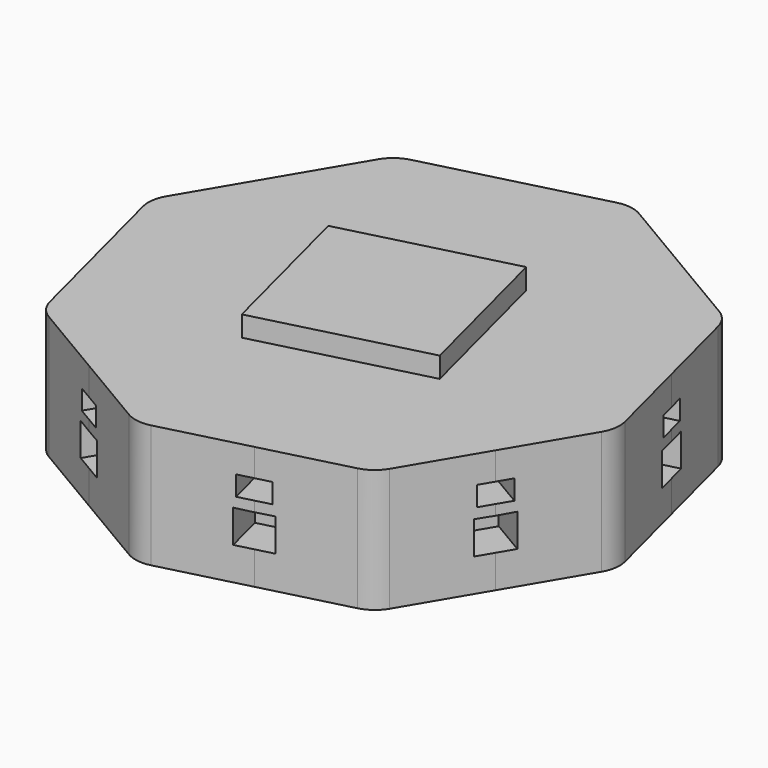
from build123d import *

# Parameters (mm, degrees)
F1_DEPTH  = 9.525
F3_DEPTH  = 6.35
F5_DEPTH  = 6.35
F7_DEPTH  = 6.35
F9_DEPTH  = 6.35
F11_DEPTH = 6.35
F13_DEPTH = 6.35
F15_DEPTH = 6.35
F17_DEPTH = 6.35
F19_DEPTH = 3.175
F20_R     = 5.08


# Not quite as in the source:
# - a feature names something its author has since deleted; it is built from what else it names


with BuildPart() as f1:
    # F0 (on Top) → F1 (new body, symmetric)
    with BuildSketch(Plane.XY):
        Polygon((-32.7905689314, 19.40073682), (-40.8266172422, 5.8184384507), (-36.9048262157, -9.4680410849), (0, 0), align=None)
        Polygon((-24.7545206205, 32.9830351893), (-32.7905689314, 19.40073682), (0, 0), (-9.4680410849, 36.9048262157), align=None)
        Polygon((-9.4680410849, 36.9048262157), (0, 0), (19.40073682, 32.7905689314), (5.8184384507, 40.8266172422), align=None)
        Polygon((19.40073682, 32.7905689314), (0, 0), (36.9048262157, 9.4680410849), (32.9830351893, 24.7545206205), align=None)
        Polygon((36.9048262157, 9.4680410849), (0, 0), (32.7905689314, -19.40073682), (40.8266172422, -5.8184384507), align=None)
        Polygon((32.7905689314, -19.40073682), (0, 0), (9.4680410849, -36.9048262157), (24.7545206205, -32.9830351893), align=None)
        Polygon((9.4680410849, -36.9048262157), (0, 0), (-19.40073682, -32.7905689314), (-5.8184384507, -40.8266172422), align=None)
        Polygon((0, 0), (-36.9048262157, -9.4680410849), (-32.9830351893, -24.7545206205), (-19.40073682, -32.7905689314), align=None)
    extrude(amount=F1_DEPTH, both=True)

    # F2 (on face) → F3 (cut)
    with BuildSketch(Plane(origin=(-36.9048262157, -9.4680410849, 0), x_dir=(0.2485050154, -0.9686306093, 0), z_dir=(-0.9686306093, -0.2485050154, 0))):
        Polygon((-2.794, 0), (-2.794, -2.521839), (-2.794, -5.043678), (2.794, -5.043678), (2.794, -2.521839), (2.794, 0), align=None)
        Polygon((-2.413, 1.556766), (0, 1.556766), (2.413, 1.556766), (2.413, 4.604766), (-2.413, 4.604766), align=None)
    extrude(amount=-F3_DEPTH, mode=Mode.SUBTRACT)

    # F4 (on face) → F5 (cut)
    with BuildSketch(Plane(origin=(-9.4680410849, 36.9048262157, 0), x_dir=(-0.9686306093, -0.2485050154, 0), z_dir=(-0.2485050154, 0.9686306093, 0))):
        Polygon((-2.794, -5.043678), (0, -5.043678), (2.794, -5.043678), (2.794, 0.036322), (0, 0), (-2.794, 0.036322), align=None)
        Polygon((-2.413, 1.593088), (0, 1.593088), (2.413, 1.593088), (2.413, 4.641088), (0, 4.641088), (-2.413, 4.641088), align=None)
    extrude(amount=-F5_DEPTH, mode=Mode.SUBTRACT)

    # F6 (on face) → F7 (cut)
    with BuildSketch(Plane(origin=(-32.7905689314, 19.40073682, 0), x_dir=(-0.5092056908, -0.8606448538, 0), z_dir=(-0.8606448538, 0.5092056908, 0))):
        Polygon((-2.413, 1.593088), (0, 1.593088), (2.413, 1.593088), (2.413, 4.641088), (0, 4.641088), (-2.413, 4.641088), align=None)
        Polygon((-2.794, -5.043678), (0, -5.043678), (2.794, -5.043678), (2.793763897, 0), (-2.793763897, 0), align=None)
    extrude(amount=-F7_DEPTH, mode=Mode.SUBTRACT)

    # F8 (on face) → F9 (cut)
    with BuildSketch(Plane(origin=(19.40073682, 32.7905689314, 0), x_dir=(-0.8606448538, 0.5092056908, 0), z_dir=(0.5092056908, 0.8606448538, 0))):
        Polygon((-2.413, 1.62941), (0, 1.62941), (2.413, 1.62941), (2.413, 4.67741), (-2.413, 4.67741), align=None)
        Polygon((-2.794, -5.043678), (0, -5.043678), (2.794, -5.043678), (2.794, 0.036322), (-2.794, 0.036322), align=None)
    extrude(amount=-F9_DEPTH, mode=Mode.SUBTRACT)

    # F10 (on face) → F11 (cut)
    with BuildSketch(Plane(origin=(36.9048262157, 9.4680410849, 0), x_dir=(-0.2485050154, 0.9686306093, 0), z_dir=(0.9686306093, 0.2485050154, 0))):
        Polygon((-2.794, -4.6912106667), (0, -4.6912106667), (2.794, -4.6912106667), (2.794, 0.3887893333), (-2.794, 0.3887893333), align=None)
        Polygon((-2.413, 1.9818773333), (0, 1.9818773333), (2.413, 1.9818773333), (2.413, 5.0298773333), (-2.413, 5.0298773333), align=None)
    extrude(amount=-F11_DEPTH, mode=Mode.SUBTRACT)

    # F12 (on face) → F13 (cut)
    with BuildSketch(Plane(origin=(32.7905689314, -19.40073682, 0), x_dir=(0.5092056908, 0.8606448538, 0), z_dir=(0.8606448538, -0.5092056908, 0))):
        Polygon((-2.7940002649, -4.4215812), (-2.649e-07, -4.4215812), (2.7939997351, -4.4215812), (2.7939997351, 0.6584188), (-2.649e-07, 0.6220968), (-2.7940002649, 0.6584188), align=None)
        Polygon((-2.4130002649, 2.2151848), (-2.649e-07, 2.2151848), (2.4129997351, 2.2151848), (2.4129997351, 5.2631848), (-2.649e-07, 5.2631848), (-2.4130002649, 5.2631848), align=None)
    extrude(amount=-F13_DEPTH, mode=Mode.SUBTRACT)

    # F14 (on face) → F15 (cut)
    with BuildSketch(Plane(origin=(9.4680410849, -36.9048262157, 0), x_dir=(0.9686306093, 0.2485050154, 0), z_dir=(0.2485050154, -0.9686306093, 0))):
        Polygon((-2.7940002649, -4.4215812), (-2.649e-07, -4.4215812), (2.7939997351, -4.4215812), (2.7939997351, 0.6584188), (-2.649e-07, 0.6220968), (-2.7940002649, 0.6584188), align=None)
        Polygon((-2.4130002649, 2.2151848), (-2.649e-07, 2.2151848), (2.4129997351, 2.2151848), (2.4129997351, 5.2631848), (-2.649e-07, 5.2631848), (-2.4130002649, 5.2631848), align=None)
    extrude(amount=-F15_DEPTH, mode=Mode.SUBTRACT)

    # F16 (on face) → F17 (cut)
    with BuildSketch(Plane(origin=(-19.40073682, -32.7905689314, 0), x_dir=(0.8606448538, -0.5092056908, 0), z_dir=(-0.5092056908, -0.8606448538, 0))):
        Polygon((-2.4130002649, 2.2151848), (-2.649e-07, 2.2151848), (2.4129997351, 2.2151848), (2.4129997351, 5.2631848), (-2.649e-07, 5.2631848), (-2.4130002649, 5.2631848), align=None)
        Polygon((-2.7940002649, -4.4215812), (-2.649e-07, -4.4215812), (2.7939997351, -4.4215812), (2.7939997351, 0.6584188), (-2.649e-07, 0.6220968), (-2.7940002649, 0.6584188), align=None)
    extrude(amount=-F17_DEPTH, mode=Mode.SUBTRACT)

    # F18 (on face) → F19 (join)
    with BuildSketch(Plane.XY.offset(9.525)):
        Polygon((-3.156013695, 12.3016087386), (-15.856013695, 9.0433866005), (-9.543986305, -15.5598308767), (3.156013695, -12.3016087386), (15.856013695, -9.0433866005), (9.543986305, 15.5598308767), align=None)
    extrude(amount=F19_DEPTH)

    # F20
    f20_edges = [f1.edges().sort_by_distance(p)[0] for p in [
        (-5.818438, -40.826617, 0),
        (24.754521, -32.983035, 0),
        (40.826617, -5.818438, 0),
        (32.983035, 24.754521, 0),
        (5.818438, 40.826617, 0),
        (-24.754521, 32.983035, 0),
        (-40.826617, 5.818438, 0),
        (-32.983035, -24.754521, 0),
    ]]
    fillet(f20_edges, radius=F20_R)


solid = f1.part
